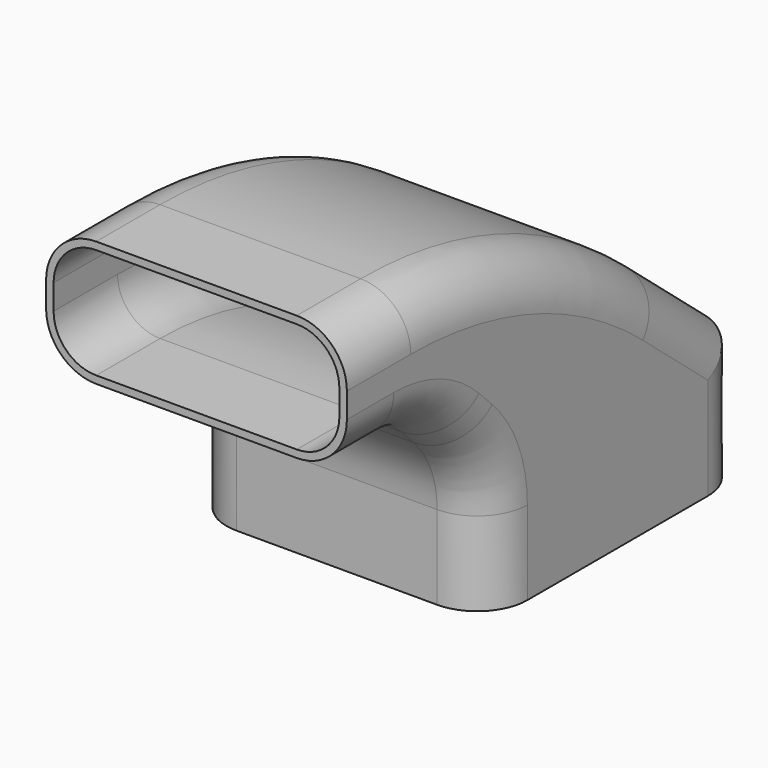
from build123d import *

# Parameters (mm, degrees)
F1_DEPTH = 152.4
F2_R     = 25.4
F3_R     = 25.4
F4_R     = 25.4
F5_R     = 25.4


# Not quite as in the source:
# - a feature names something its author has since deleted; it is built from what else it names


with BuildPart() as f1:
    # F0 (on Right) → F1 (new body)
    with BuildSketch(Plane.YZ):
        with BuildLine():
            Line((0, -63.5), (0, 0))
            Line((0, 0), (-50.2625516508, 42.1752885522))
            ThreePointArc((-50.2625516508, 42.1752885522), (-126.6574881065, 86.2819256796), (-213.5306045112, 101.6))
            Line((-213.5306045112, 101.6), (-254, 101.6))
            Line((-254, 101.6), (-254, 38.1))
            Line((-254, 38.1), (-224.2420489686, 38.1))
            ThreePointArc((-224.2420489686, 38.1), (-204.8017306044, 34.2330802516), (-188.3210244843, 23.2210244843))
            Line((-188.3210244843, 23.2210244843), (-179.9789755157, 14.8789755157))
            ThreePointArc((-179.9789755157, 14.8789755157), (-168.9669197484, -1.6017306044), (-165.1, -21.0420489686))
            Line((-165.1, -21.0420489686), (-165.1, -63.5))
            Line((-165.1, -63.5), (0, -63.5))
        make_face()
    extrude(amount=F1_DEPTH)

    # F2
    f2_edges = [f1.edges().sort_by_distance(p)[0] for p in [
        (0, -233.765302, 101.6),
        (0, 0, -31.75),
    ]]
    fillet(f2_edges, radius=F2_R)

    # F3
    f3_edges = [f1.edges().sort_by_distance(p)[0] for p in [
        (0, -165.1, -42.271024),
    ]]
    fillet(f3_edges, radius=F3_R)

    # F4
    f4_edges = [f1.edges().sort_by_distance(p)[0] for p in [
        (152.4, -165.1, -42.271024),
    ]]
    fillet(f4_edges, radius=F4_R)

    # F5
    f5_edges = [f1.edges().sort_by_distance(p)[0] for p in [
        (152.4, -233.765302, 101.6),
        (152.4, 0, -31.75),
    ]]
    fillet(f5_edges, radius=F5_R)

    # F9: sweep along a path in F8
    with BuildLine(Plane.YZ.offset(76.2)) as f9_path:
        Line((-254, 69.85), (-213.5306045112, 69.85))
        ThreePointArc((-213.5306045112, 69.85), (-137.5166276571, 56.4466849697), (-70.6710582584, 17.8533774832))
        Line((-70.6710582584, 17.8533774832), (74.6758873088, -104.1071909349))
    # F6 (on face) → F9 (sweep, cut)
    with BuildSketch(Plane.XZ.offset(254)):
        with BuildLine():
            Line((25.4, 41.91), (127, 41.91))
            ThreePointArc((127, 41.91), (142.2664354058, 48.2335645942), (148.59, 63.5))
            Line((148.59, 63.5), (148.59, 76.2))
            ThreePointArc((148.59, 76.2), (142.2664354058, 91.4664354058), (127, 97.79))
            Line((127, 97.79), (25.4, 97.79))
            ThreePointArc((25.4, 97.79), (10.1335645942, 91.4664354058), (3.81, 76.2))
            Line((3.81, 76.2), (3.81, 63.5))
            ThreePointArc((3.81, 63.5), (10.1335645942, 48.2335645942), (25.4, 41.91))
        make_face()
    sweep(path=f9_path.line, mode=Mode.SUBTRACT)


solid = f1.part
